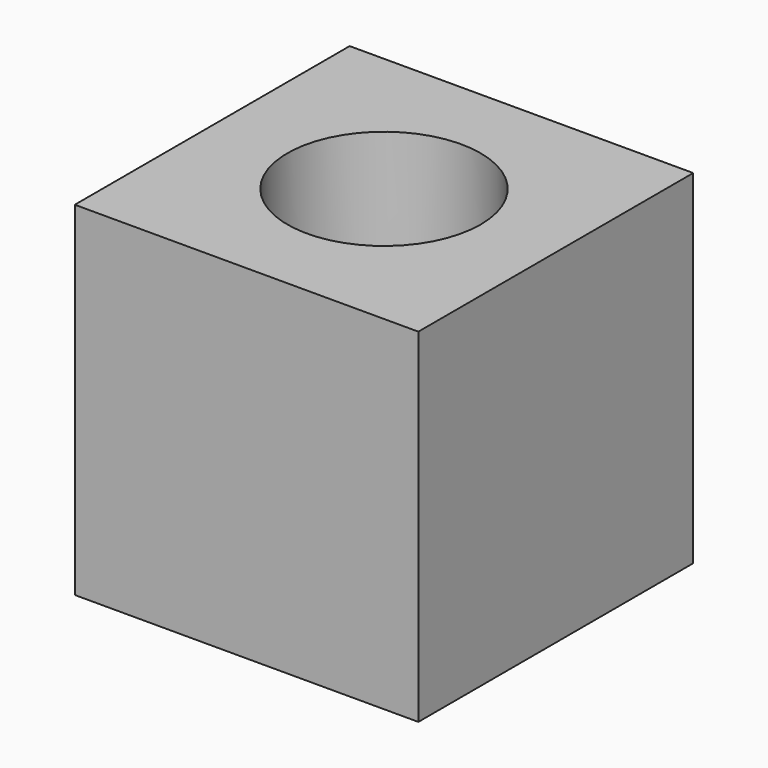
from build123d import *

# Parameters (mm, degrees)
F0_W           = 20
F0_H           = 20
F1_DEPTH       = 20
F3_D           = 6.3
F3_CBORE_D     = 11.25
F3_CBORE_DEPTH = 6
F5_DEPTH       = 7
F6_TEXT_SIZE   = 7.6795274137
F7_DEPTH       = 1


# Not quite as in the source:
# - Text() gives the source's letters only with a copy of the font that has no kerning and outlines rounded to 1/6400 em; it was checked with that copy


with BuildPart() as f1:
    # F0 (on Top) → F1 (new body)
    with BuildSketch(Plane.XY):
        with Locations((10, 10)):
            Rectangle(F0_W, F0_H)
    extrude(amount=F1_DEPTH)

    # F3 (through all)
    with Locations(Plane.XY.offset(20)):
        with Locations((10, 10)):
            CounterBoreHole(F3_D / 2, F3_CBORE_D / 2, F3_CBORE_DEPTH)

    # F4 (on face) → F5 (cut)
    with BuildSketch(Plane(origin=(0, 0, 0), x_dir=(1, 0, 0), z_dir=(0, 0, -1))):
        with BuildLine():
            ThreePointArc((14.3344572498, -12.5024998201), (14.8344587875, -11.2953892204), (15.005, -10))
            ThreePointArc((15.005, -10), (14.8344587875, -8.7046107796), (14.3344572498, -7.4975001799))
            ThreePointArc((14.3344572498, -7.4975001799), (12.5025000899, -5.665542906), (10, -4.995))
            ThreePointArc((10, -4.995), (7.4974999957, -5.6655428565), (5.6655428491, -7.4975000086))
            ThreePointArc((5.6655428491, -7.4975000086), (4.995, -9.999999955), (5.6655428041, -12.5024999135))
            ThreePointArc((5.6655428041, -12.5024999135), (7.4974999567, -14.334457121), (10, -15.005))
            ThreePointArc((10, -15.005), (12.5025000899, -14.334457094), (14.3344572498, -12.5024998201))
        make_face()
        with BuildLine():
            ThreePointArc((14.3344572498, -7.4975001799), (14.8344587875, -8.7046107796), (15.005, -10))
            ThreePointArc((15.005, -10), (14.8344587875, -11.2953892204), (14.3344572498, -12.5024998201))
            Line((14.3344572498, -12.5024998201), (15.7792761946, -10))
            Line((15.7792761946, -10), (14.3344572498, -7.4975001799))
        make_face()
        with BuildLine():
            ThreePointArc((10, -4.995), (12.5025000899, -5.665542906), (14.3344572498, -7.4975001799))
            Line((14.3344572498, -7.4975001799), (12.8896380973, -4.995))
            Line((12.8896380973, -4.995), (10, -4.995))
        make_face()
        with BuildLine():
            Line((12.8896380973, -15.005), (14.3344572498, -12.5024998201))
            ThreePointArc((14.3344572498, -12.5024998201), (12.5025000899, -14.334457094), (10, -15.005))
            Line((10, -15.005), (12.8896380973, -15.005))
        make_face()
        with BuildLine():
            ThreePointArc((5.6655428491, -7.4975000086), (7.4974999957, -5.6655428565), (10, -4.995))
            Line((10, -4.995), (7.1103619027, -4.995))
            Line((7.1103619027, -4.995), (5.6655428491, -7.4975000086))
        make_face()
        with BuildLine():
            Line((7.1103619027, -15.005), (10, -15.005))
            ThreePointArc((10, -15.005), (7.4974999567, -14.334457121), (5.6655428041, -12.5024999135))
            Line((5.6655428041, -12.5024999135), (7.1103619027, -15.005))
        make_face()
        with BuildLine():
            ThreePointArc((5.6655428041, -12.5024999135), (4.995, -9.999999955), (5.6655428491, -7.4975000086))
            Line((5.6655428491, -7.4975000086), (4.2207238054, -10))
            Line((4.2207238054, -10), (5.6655428041, -12.5024999135))
        make_face()
    extrude(amount=-F5_DEPTH, mode=Mode.SUBTRACT)

    # F6 (on face) → F7 (join)
    with BuildSketch(Plane(origin=(0, 20, 0), x_dir=(-1, 0, 0), z_dir=(0, 1, 0))):
        with Locations((-17.5, 2.5)):
            Text('LFB', F6_TEXT_SIZE, font='Open Sans', text_align=(TextAlign.LEFT, TextAlign.BOTTOM))
    extrude(amount=F7_DEPTH)


solid = f1.part
